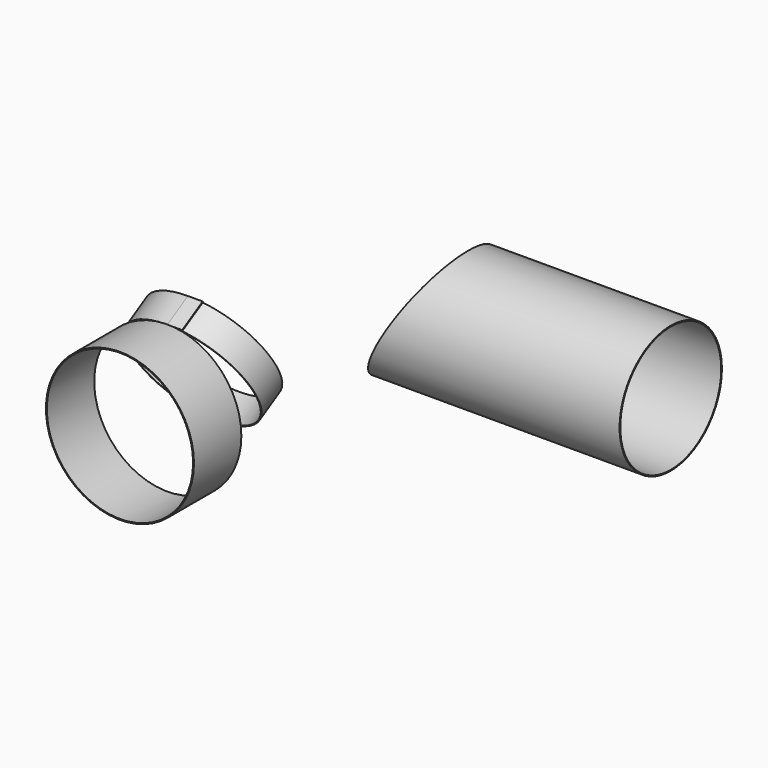
from build123d import *

# Parameters (mm, degrees)
F0_R     = 125
F0_R_2   = 123.5
F1_DEPTH = 100
F4_DEPTH = 25
F5_R     = 108
F5_R_2   = 106.5
F6_DEPTH = 500
F8_DEPTH = 600


with BuildPart() as f1:
    # F0 (on Front) → F1 (new body)
    with BuildSketch(Plane.XZ):
        Circle(F0_R)
        Circle(F0_R_2, mode=Mode.SUBTRACT)
    extrude(amount=F1_DEPTH)


with BuildPart() as f3:
    # F2 (on Right) → F3 (revolve)
    with BuildSketch(Plane.YZ):
        Polygon((43.3012701892, 149.707658145), (0, 124.707658145), (0.75, 123.4086200393), (44.0512701892, 148.4086200393), align=None)
    revolve(axis=Axis((0, 48.6506350946, 28.0884572681), (0, 0.8660254038, 0.5)))

    # F2 (on Right) → F4 (join)
    with BuildSketch(Plane.YZ):
        Polygon((43.3012701892, 149.707658145), (0, 124.707658145), (0.75, 123.4086200393), (44.0512701892, 148.4086200393), align=None)
    extrude(amount=F4_DEPTH)


with BuildPart() as f6:
    # F5 (on Right) → F6 (new body)
    with BuildSketch(Plane.YZ):
        with Locations((437.6462212987, 0)):
            Circle(F5_R)
        with Locations((437.6462212987, 0)):
            Circle(F5_R_2, mode=Mode.SUBTRACT)
    extrude(amount=F6_DEPTH)

    # F7 (on Front) → F8 (cut)
    with BuildSketch(Plane.XZ):
        Polygon((-296.155548444, 26.1171597825), (8.8311323739, -149.966982487), (209.2771804602, 197.2157569749), (-95.7095003577, 373.2998992443), align=None)
    extrude(amount=-F8_DEPTH, mode=Mode.SUBTRACT)


solid = Compound([f1.part, f3.part, f6.part])
